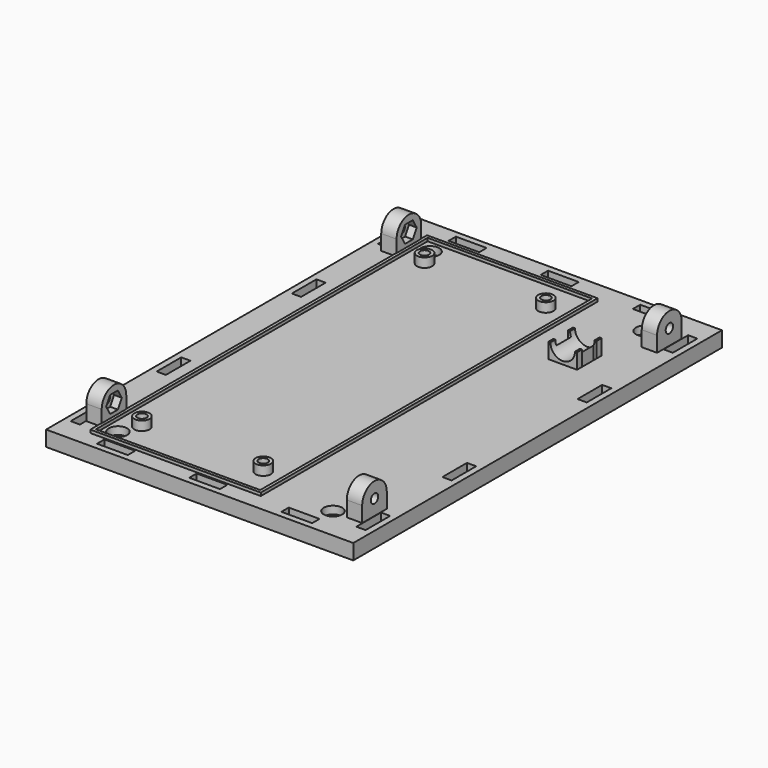
from build123d import *

# Parameters (mm, degrees)
F0_W      = 100
F0_H      = 150
F1_DEPTH  = 5
F2_R      = 1.5
F3_DEPTH  = 25
F4_R      = 2.5
F4_R_2    = 1.5
F5_DEPTH  = 3
F6_R      = 2.75
F7_DEPTH  = 2.5
F8_W      = 3
F8_H      = 10
F8_W_2    = 5
F8_H_2    = 3
F8_W_3    = 10
F9_DEPTH  = 25
F10_W     = 55.5
F10_H     = 137
F10_W_2   = 53.5
F10_H_2   = 135
F11_DEPTH = 1
F12_W     = 1
F12_H     = 6
F13_DEPTH = 5
F14_DEPTH = 12.5
F15_R     = 4
F16_DEPTH = 25
F17_W     = 9.35
F17_H     = 6
F18_DEPTH = 2
F19_W     = 5
F19_H     = 10
F20_DEPTH = 12
F21_R     = 1.5
F22_DEPTH = 150
F24_DEPTH = 2.5
F26_DEPTH = 2.5
F28_DEPTH = 150
F29_R     = 1.5
F30_DEPTH = 25
F31_R     = 3
F32_DEPTH = 2.5


# Not quite as in the source:
# - a feature names something its author has since deleted; it is built from what else it names


with BuildPart() as f1:
    # F0 (on Top) → F1 (new body)
    with BuildSketch(Plane.XY):
        Rectangle(F0_W, F0_H)
    extrude(amount=F1_DEPTH)

    # F2 (on face) → F3 (cut)
    with BuildSketch(Plane.XY.offset(5)):
        with Locations((-32, 56.5)):
            Circle(F2_R)
        with Locations((7.5, 56.5)):
            Circle(F2_R)
        with Locations((-32, -58.5)):
            Circle(F2_R)
        with Locations((7.5, -58.5)):
            Circle(F2_R)
    extrude(amount=-F3_DEPTH, mode=Mode.SUBTRACT)

    # F4 (on face) → F5 (join)
    with BuildSketch(Plane.XY.offset(5)):
        with Locations((-32, -58.5)):
            Circle(F4_R)
        with Locations((-32, -58.5)):
            Circle(F4_R_2, mode=Mode.SUBTRACT)
        with Locations((7.5, -58.5)):
            Circle(F4_R)
        with Locations((7.5, -58.5)):
            Circle(F4_R_2, mode=Mode.SUBTRACT)
        with Locations((7.5, 56.5)):
            Circle(F4_R)
        with Locations((7.5, 56.5)):
            Circle(F4_R_2, mode=Mode.SUBTRACT)
        with Locations((-32, 56.5)):
            Circle(F4_R)
        with Locations((-32, 56.5)):
            Circle(F4_R_2, mode=Mode.SUBTRACT)
    extrude(amount=F5_DEPTH)

    # F6 (on face) → F7 (cut)
    with BuildSketch(Plane(origin=(0, 0, 0), x_dir=(1, 0, 0), z_dir=(0, 0, -1))):
        with Locations((-32, 58.5)):
            Circle(F6_R)
        with Locations((7.5, 58.5)):
            Circle(F6_R)
        with Locations((-32, -56.5)):
            Circle(F6_R)
        with Locations((7.5, -56.5)):
            Circle(F6_R)
    extrude(amount=-F7_DEPTH, mode=Mode.SUBTRACT)

    # F8 (on face) → F9 (cut)
    with BuildSketch(Plane.XY.offset(5)):
        with Locations((-46.5, 62.5)):
            Rectangle(F8_W, F8_H)
        with Locations((-46.5, 27.5)):
            Rectangle(F8_W, F8_H)
        with Locations((-46.5, -27.5)):
            Rectangle(F8_W, F8_H)
        with Locations((-46.5, -62.5)):
            Rectangle(F8_W, F8_H)
        with Locations((2.5, 71.5)):
            Rectangle(F8_W_2, F8_H_2)
        with Locations((-2.5, 71.5)):
            Rectangle(F8_W_2, F8_H_2)
        with Locations((2.5, -71.5)):
            Rectangle(F8_W_2, F8_H_2)
        with Locations((-2.5, -71.5)):
            Rectangle(F8_W_2, F8_H_2)
        with Locations((46.5, 62.5)):
            Rectangle(F8_W, F8_H)
        with Locations((46.5, -62.5)):
            Rectangle(F8_W, F8_H)
        with Locations((46.5, -27.5)):
            Rectangle(F8_W, F8_H)
        with Locations((46.5, 27.5)):
            Rectangle(F8_W, F8_H)
        with Locations((-30, 71.5)):
            Rectangle(F8_W_3, F8_H_2)
        with Locations((30, 71.5)):
            Rectangle(F8_W_3, F8_H_2)
        with Locations((30, -71.5)):
            Rectangle(F8_W_3, F8_H_2)
        with Locations((-30, -71.5)):
            Rectangle(F8_W_3, F8_H_2)
    extrude(amount=-F9_DEPTH, mode=Mode.SUBTRACT)

    # F10 (on face) → F11 (join)
    with BuildSketch(Plane.XY.offset(5)):
        with Locations((-12.25, -1)):
            Rectangle(F10_W, F10_H)
        with Locations((-12.25, -1)):
            Rectangle(F10_W_2, F10_H_2, mode=Mode.SUBTRACT)
    extrude(amount=F11_DEPTH)

    # F12 (on face) → F13 (join)
    with BuildSketch(Plane.XY.offset(5)):
        Polygon((34.85, 45), (25.5, 45), (25.5, 43), (26.5, 43), (26.5, 37), (25.5, 37), (25.5, 35), (34.85, 35), (34.85, 37), (33.85, 37), (33.85, 43), (34.85, 43), align=None)
        with Locations((26, 40)):
            Rectangle(F12_W, F12_H)
        with Locations((34.35, 40)):
            Rectangle(F12_W, F12_H)
    extrude(amount=F13_DEPTH)

    # F12 (on face) → F14 (cut, symmetric)
    with BuildSketch(Plane.XY.offset(5)):
        with Locations((34.35, 40)):
            Rectangle(F12_W, F12_H)
        with Locations((26, 40)):
            Rectangle(F12_W, F12_H)
    extrude(amount=F14_DEPTH, both=True, mode=Mode.SUBTRACT)

    # F15 (on face) → F16 (cut)
    with BuildSketch(Plane.XZ.offset(-35)):
        with Locations((30.175, 10)):
            Circle(F15_R)
    extrude(amount=-F16_DEPTH, mode=Mode.SUBTRACT)

    # F17 (on face) → F18 (cut)
    with BuildSketch(Plane(origin=(0, 0, 0), x_dir=(1, 0, 0), z_dir=(0, 0, -1))):
        with Locations((30.175, -40)):
            Rectangle(F17_W, F17_H)
    extrude(amount=-F18_DEPTH, mode=Mode.SUBTRACT)

    # F19 (on face) → F20 (join)
    with BuildSketch(Plane.XY.offset(5)):
        with Locations((42.4, 60)):
            Rectangle(F19_W, F19_H)
        with Locations((-42.4, 60)):
            Rectangle(F19_W, F19_H)
        with Locations((-42.4, -60)):
            Rectangle(F19_W, F19_H)
        with Locations((42.4, -60)):
            Rectangle(F19_W, F19_H)
    extrude(amount=F20_DEPTH)

    # F21 (on face) → F22 (cut)
    with BuildSketch(Plane.YZ.offset(44.9)):
        with Locations((-60, 10)):
            Circle(F21_R)
        with Locations((60, 10)):
            Circle(F21_R)
    extrude(amount=-F22_DEPTH, mode=Mode.SUBTRACT)

    # F23 (on face) → F24 (cut)
    with BuildSketch(Plane(origin=(39.9, 0, 0), x_dir=(0, -1, 0), z_dir=(-1, 0, 0))):
        Polygon((-58.4122867597, 12.75), (-61.5877132403, 12.75), (-63.1754264805, 10), (-61.5877132403, 7.25), (-58.4122867597, 7.25), (-56.8245735195, 10), align=None)
        Polygon((61.5877132403, 7.25), (63.1754264805, 10), (61.5877132403, 12.75), (58.4122867597, 12.75), (56.8245735195, 10), (58.4122867597, 7.25), align=None)
    extrude(amount=-F24_DEPTH, mode=Mode.SUBTRACT)

    # F25 (on face) → F26 (cut)
    with BuildSketch(Plane.YZ.offset(-39.9)):
        Polygon((-58.4122867597, 12.75), (-61.5877132403, 12.75), (-63.1754264805, 10), (-61.5877132403, 7.25), (-58.4122867597, 7.25), (-56.8245735195, 10), align=None)
        Polygon((61.5877132403, 7.25), (63.1754264805, 10), (61.5877132403, 12.75), (58.4122867597, 12.75), (56.8245735195, 10), (58.4122867597, 7.25), align=None)
    extrude(amount=-F26_DEPTH, mode=Mode.SUBTRACT)

    # F27 (on face) → F28 (cut)
    with BuildSketch(Plane.YZ.offset(44.9)):
        with BuildLine():
            ThreePointArc((-65, 10), (-60, 15), (-55, 10))
            Line((-55, 10), (-55, 17))
            Line((-55, 17), (-65, 17))
            Line((-65, 17), (-65, 10))
        make_face()
        with BuildLine():
            ThreePointArc((55, 10), (60, 15), (65, 10))
            Line((65, 10), (65, 17))
            Line((65, 17), (55, 17))
            Line((55, 17), (55, 10))
        make_face()
    extrude(amount=-F28_DEPTH, mode=Mode.SUBTRACT)

    # F29 (on face) → F30 (cut)
    with BuildSketch(Plane.XY.offset(5)):
        with Locations((-35, 62.5)):
            Circle(F29_R)
        with Locations((35, 62.5)):
            Circle(F29_R)
        with Locations((-35, -64.5)):
            Circle(F29_R)
        with Locations((35, -64.5)):
            Circle(F29_R)
    extrude(amount=-F30_DEPTH, mode=Mode.SUBTRACT)

    # F31 (on face) → F32 (cut)
    with BuildSketch(Plane.XY.offset(5)):
        with Locations((35, -64.5)):
            Circle(F31_R)
        with Locations((35, 62.5)):
            Circle(F31_R)
        with Locations((-35, 62.5)):
            Circle(F31_R)
        with Locations((-35, -64.5)):
            Circle(F31_R)
    extrude(amount=-F32_DEPTH, mode=Mode.SUBTRACT)


solid = f1.part
